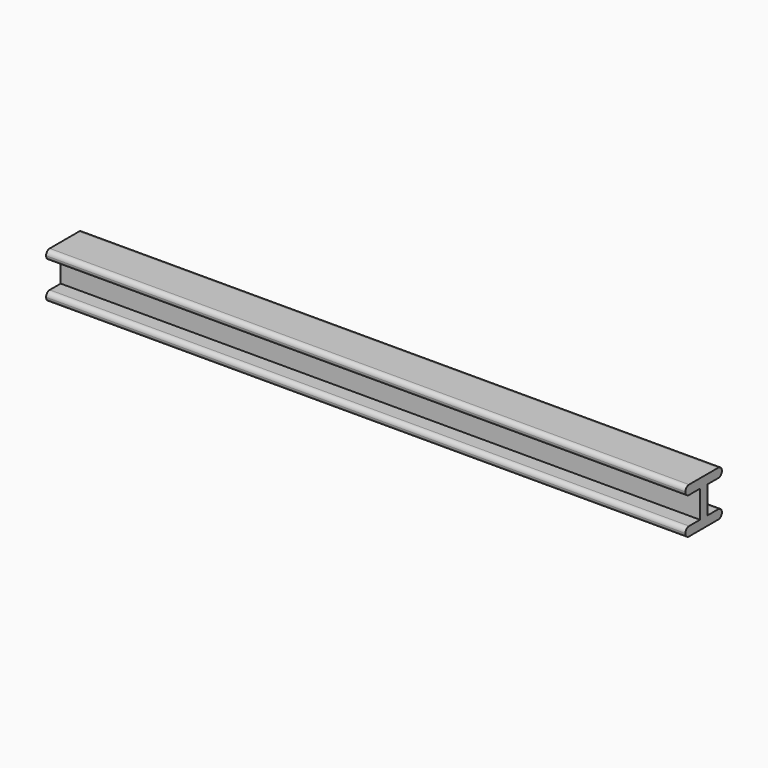
from build123d import *

# Parameters (mm, degrees)
F0_W     = 177.8
F0_H     = 12.7
F1_DEPTH = 12.7
F2_R     = 1.27
F3_W     = 5.08
F3_H     = 7.62
F4_DEPTH = 177.8
F5_R     = 1.26999


# Not quite as in the source:
# - a fillet or chamfer is up to 0.001 mm smaller than in the source, because OpenCascade refuses the exact size


with BuildPart() as f1:
    # F0 (on Top) → F1 (new body)
    with BuildSketch(Plane.XY):
        Rectangle(F0_W, F0_H)
    extrude(amount=F1_DEPTH)

    # F2
    f2_edges = [f1.edges().sort_by_distance(p)[0] for p in [
        (0, 6.35, 12.7),
        (0, -6.35, 12.7),
        (0, 6.35, 0),
        (0, -6.35, 0),
    ]]
    fillet(f2_edges, radius=F2_R)

    # F3 (on face) → F4 (cut)
    with BuildSketch(Plane.YZ.offset(88.9)):
        with Locations((-3.81, 6.35)):
            Rectangle(F3_W, F3_H)
        with Locations((3.81, 6.35)):
            Rectangle(F3_W, F3_H)
    extrude(amount=-F4_DEPTH, mode=Mode.SUBTRACT)

    # F5 (radius 1.27 in the source; OpenCascade refuses exactly that, so slightly less here)
    f5_edges = [f1.edges().sort_by_distance(p)[0] for p in [
        (0, -6.35, 10.16),
        (0, -6.35, 2.54),
        (0, 6.35, 2.54),
        (0, 6.35, 10.16),
    ]]
    fillet(f5_edges, radius=F5_R)


solid = f1.part
